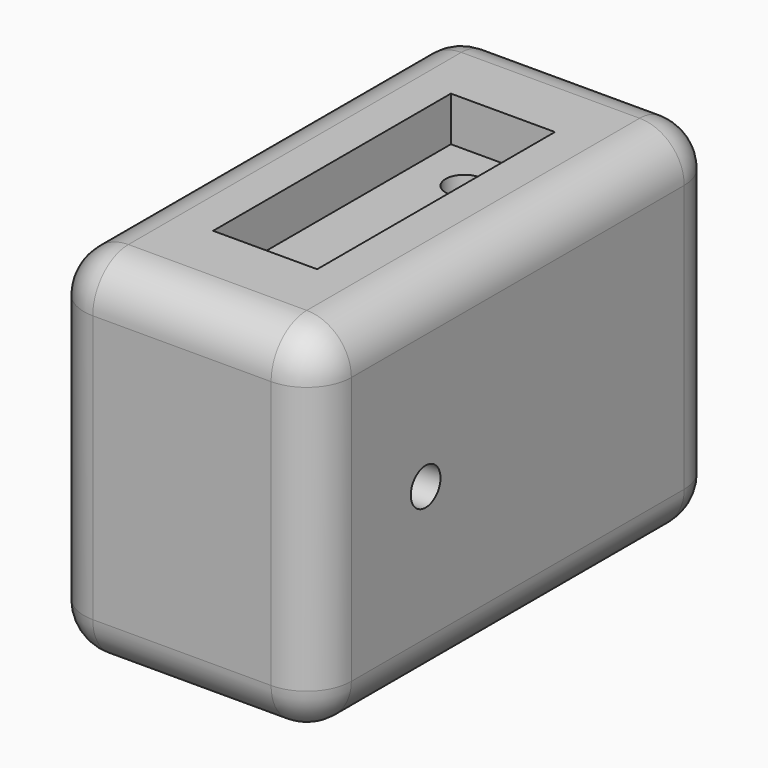
from build123d import *

# Parameters (mm, degrees)
F0_W         = 18
F0_H         = 24
F1_DEPTH     = 34
F2_W         = 25
F2_H         = 13
F2_R         = 1.25
F3_DEPTH     = 16
F4_W         = 7
F4_H         = 20
F5_DEPTH     = 3
F6_R         = 1.25
F7_DEPTH     = 4
F8_T1_DEPTH  = 28
F8_T3_DEPTH  = 18
F8_T5_DEPTH  = 12
F8_S9_W      = 3
F8_S9_H      = 3
F8_T10_DEPTH = 3
F8_S15_W     = 3
F8_S15_H     = 3
F8_T16_DEPTH = 3
F8_S21_W     = 3
F8_S21_H     = 3
F8_T22_DEPTH = 3
F8_S27_W     = 3
F8_S27_H     = 3
F8_T28_DEPTH = 3
F8_S33_W     = 3
F8_S33_H     = 3
F8_T34_DEPTH = 3
F8_S39_W     = 3
F8_S39_H     = 3
F8_T40_DEPTH = 3
F8_S45_W     = 3
F8_S45_H     = 3
F8_T46_DEPTH = 3
F8_S51_W     = 3
F8_S51_H     = 3
F8_T52_DEPTH = 3
F9_R         = 3.5
F10_DEPTH    = 19
F11_R        = 1.25
F12_DEPTH    = 18.0010001


# Not quite as in the source:
# - a fillet or chamfer that OpenCascade refuses, or shapes differently, is made with other operations: its cross-section is extruded or revolved along the edge and cut away or added


with BuildPart() as f1:
    # F0 (on Front) → F1 (new body)
    with BuildSketch(Plane.XZ):
        with Locations((-10.5989521787, -5.2339873202)):
            Rectangle(F0_W, F0_H)
    extrude(amount=F1_DEPTH)

    # F2 (on face) → F3 (cut)
    with BuildSketch(Plane(origin=(-19.5989521787, 0, 0), x_dir=(0, -1, 0), z_dir=(-1, 0, 0))):
        with Locations((17, -7.2339873202)):
            Rectangle(F2_W, F2_H)
        with Locations((2.25, -7.2339873202)):
            Circle(F2_R)
        with Locations((31.75, -7.2339873202)):
            Circle(F2_R)
    extrude(amount=-F3_DEPTH, mode=Mode.SUBTRACT)

    # F4 (on face) → F5 (cut)
    with BuildSketch(Plane.XY.offset(6.7660126798)):
        with Locations((-10.5989521787, -17)):
            Rectangle(F4_W, F4_H)
    extrude(amount=-F5_DEPTH, mode=Mode.SUBTRACT)

    # F6 (on face) → F7 (cut)
    with BuildSketch(Plane.XY.offset(3.7660126798)):
        with Locations((-10.5989521787, -10.25)):
            Circle(F6_R)
        with Locations((-10.5989521787, -23.75)):
            Circle(F6_R)
    extrude(amount=-F7_DEPTH, mode=Mode.SUBTRACT)

    # F8: fillet of radius 3 on 12 edges, made by hand

    # F8_s2 → F8_t1 (cut)
    with BuildSketch(Plane.XZ.offset(3)):
        with BuildLine():
            ThreePointArc((-19.5989521787, 3.7660126798), (-18.7202725222, 5.8873330233), (-16.5989521787, 6.7660126798))
            Line((-16.5989521787, 6.7660126798), (-19.5989521787, 6.7660126798))
            Line((-19.5989521787, 6.7660126798), (-19.5989521787, 3.7660126798))
        make_face()
        with BuildLine():
            ThreePointArc((-16.5989521787, -17.2339873202), (-18.7202725222, -16.3553076638), (-19.5989521787, -14.2339873202))
            Line((-19.5989521787, -14.2339873202), (-19.5989521787, -17.2339873202))
            Line((-19.5989521787, -17.2339873202), (-16.5989521787, -17.2339873202))
        make_face()
        with BuildLine():
            ThreePointArc((-4.5989521787, -17.2339873202), (-2.4776318351, -16.3553076638), (-1.5989521787, -14.2339873202))
            Line((-1.5989521787, -14.2339873202), (-1.5989521787, -17.2339873202))
            Line((-1.5989521787, -17.2339873202), (-4.5989521787, -17.2339873202))
        make_face()
        with BuildLine():
            ThreePointArc((-1.5989521787, 3.7660126798), (-2.4776318351, 5.8873330233), (-4.5989521787, 6.7660126798))
            Line((-4.5989521787, 6.7660126798), (-1.5989521787, 6.7660126798))
            Line((-1.5989521787, 6.7660126798), (-1.5989521787, 3.7660126798))
        make_face()
    extrude(amount=F8_T1_DEPTH, mode=Mode.SUBTRACT)

    # F8_s4 → F8_t3 (cut)
    with BuildSketch(Plane.XY.offset(-14.2339873202)):
        with BuildLine():
            ThreePointArc((-19.5989521787, -31), (-18.7202725222, -33.1213203436), (-16.5989521787, -34))
            Line((-16.5989521787, -34), (-19.5989521787, -34))
            Line((-19.5989521787, -34), (-19.5989521787, -31))
        make_face()
        with BuildLine():
            ThreePointArc((-1.5989521787, -31), (-2.4776318351, -33.1213203436), (-4.5989521787, -34))
            Line((-4.5989521787, -34), (-1.5989521787, -34))
            Line((-1.5989521787, -34), (-1.5989521787, -31))
        make_face()
        with BuildLine():
            ThreePointArc((-19.5989521787, -3), (-18.7202725222, -0.8786796564), (-16.5989521787, 0))
            Line((-16.5989521787, 0), (-19.5989521787, 0))
            Line((-19.5989521787, 0), (-19.5989521787, -3))
        make_face()
        with BuildLine():
            ThreePointArc((-1.5989521787, -3), (-2.4776318351, -0.8786796564), (-4.5989521787, 0))
            Line((-4.5989521787, 0), (-1.5989521787, 0))
            Line((-1.5989521787, 0), (-1.5989521787, -3))
        make_face()
    extrude(amount=F8_T3_DEPTH, mode=Mode.SUBTRACT)

    # F8_s6 → F8_t5 (cut)
    with BuildSketch(Plane.YZ.offset(-16.5989521787)):
        with BuildLine():
            ThreePointArc((-31, -17.2339873202), (-33.1213203436, -16.3553076638), (-34, -14.2339873202))
            Line((-34, -14.2339873202), (-34, -17.2339873202))
            Line((-34, -17.2339873202), (-31, -17.2339873202))
        make_face()
        with BuildLine():
            ThreePointArc((0, 3.7660126798), (-0.8786796564, 5.8873330233), (-3, 6.7660126798))
            Line((-3, 6.7660126798), (0, 6.7660126798))
            Line((0, 6.7660126798), (0, 3.7660126798))
        make_face()
        with BuildLine():
            ThreePointArc((-34, 3.7660126798), (-33.1213203436, 5.8873330233), (-31, 6.7660126798))
            Line((-31, 6.7660126798), (-34, 6.7660126798))
            Line((-34, 6.7660126798), (-34, 3.7660126798))
        make_face()
        with BuildLine():
            ThreePointArc((-3, -17.2339873202), (-0.8786796564, -16.3553076638), (0, -14.2339873202))
            Line((0, -14.2339873202), (0, -17.2339873202))
            Line((0, -17.2339873202), (-3, -17.2339873202))
        make_face()
    extrude(amount=F8_T5_DEPTH, mode=Mode.SUBTRACT)


with BuildPart() as f8_tool8:
    # F8_s9 → F8_t10 (new body)
    with BuildSketch(Plane.YZ.offset(-16.5989521787)):
        with Locations((-1.5, 5.2660126798)):
            Rectangle(F8_S9_W, F8_S9_H)
    extrude(amount=-F8_T10_DEPTH)

    # F8_s11 → F8_t12 (revolve, cut)
    with BuildSketch(Plane(origin=(-16.5989521787, -3, 3.7660126798), x_dir=(0, -0.7071067812, -0.7071067812), z_dir=(0, 0.7071067812, -0.7071067812))):
        with BuildLine():
            ThreePointArc((0, -3), (3, 0), (0, 3))
            Line((0, 3), (0, -3))
        make_face()
    revolve(axis=Axis((-16.5989521787, -3, 3.7660126798), (-1, 0, 0)), mode=Mode.SUBTRACT)


with BuildPart() as f1_1:
    add(f1.part)

    # F8_t7: cut F8_tool8
    add(f8_tool8.part, mode=Mode.SUBTRACT)


with BuildPart() as f8_tool14:
    # F8_s15 → F8_t16 (new body)
    with BuildSketch(Plane.YZ.offset(-16.5989521787)):
        with Locations((-32.5, 5.2660126798)):
            Rectangle(F8_S15_W, F8_S15_H)
    extrude(amount=-F8_T16_DEPTH)

    # F8_s17 → F8_t18 (revolve, cut)
    with BuildSketch(Plane(origin=(-16.5989521787, -31, 3.7660126798), x_dir=(0, 0.7071067812, -0.7071067812), z_dir=(0, 0.7071067812, 0.7071067812))):
        with BuildLine():
            ThreePointArc((0, -3), (3, 0), (0, 3))
            Line((0, 3), (0, -3))
        make_face()
    revolve(axis=Axis((-16.5989521787, -31, 3.7660126798), (-1, 0, 0)), mode=Mode.SUBTRACT)


with BuildPart() as f1_2:
    add(f1_1.part)

    # F8_t13: cut F8_tool14
    add(f8_tool14.part, mode=Mode.SUBTRACT)


with BuildPart() as f8_tool20:
    # F8_s21 → F8_t22 (new body)
    with BuildSketch(Plane.XY.offset(-14.2339873202)):
        with Locations((-18.0989521787, -32.5)):
            Rectangle(F8_S21_W, F8_S21_H)
    extrude(amount=-F8_T22_DEPTH)

    # F8_s23 → F8_t24 (revolve, cut)
    with BuildSketch(Plane(origin=(-16.5989521787, -31, -14.2339873202), x_dir=(0.7071067812, 0.7071067812, 0), z_dir=(-0.7071067812, 0.7071067812, 0))):
        with BuildLine():
            ThreePointArc((0, -3), (3, 0), (0, 3))
            Line((0, 3), (0, -3))
        make_face()
    revolve(axis=Axis((-16.5989521787, -31, -14.2339873202), (0, 0, -1)), mode=Mode.SUBTRACT)


with BuildPart() as f1_3:
    add(f1_2.part)

    # F8_t19: cut F8_tool20
    add(f8_tool20.part, mode=Mode.SUBTRACT)


with BuildPart() as f8_tool26:
    # F8_s27 → F8_t28 (new body)
    with BuildSketch(Plane.XY.offset(-14.2339873202)):
        with Locations((-3.0989521787, -32.5)):
            Rectangle(F8_S27_W, F8_S27_H)
    extrude(amount=-F8_T28_DEPTH)

    # F8_s29 → F8_t30 (revolve, cut)
    with BuildSketch(Plane(origin=(-4.5989521787, -31, -14.2339873202), x_dir=(-0.7071067812, 0.7071067812, 0), z_dir=(-0.7071067812, -0.7071067812, 0))):
        with BuildLine():
            ThreePointArc((0, -3), (3, 0), (0, 3))
            Line((0, 3), (0, -3))
        make_face()
    revolve(axis=Axis((-4.5989521787, -31, -14.2339873202), (0, 0, -1)), mode=Mode.SUBTRACT)


with BuildPart() as f1_4:
    add(f1_3.part)

    # F8_t25: cut F8_tool26
    add(f8_tool26.part, mode=Mode.SUBTRACT)


with BuildPart() as f8_tool32:
    # F8_s33 → F8_t34 (new body)
    with BuildSketch(Plane.YZ.offset(-4.5989521787)):
        with Locations((-32.5, 5.2660126798)):
            Rectangle(F8_S33_W, F8_S33_H)
    extrude(amount=F8_T34_DEPTH)

    # F8_s35 → F8_t36 (revolve, cut)
    with BuildSketch(Plane(origin=(-4.5989521787, -31, 3.7660126798), x_dir=(0, 0.7071067812, -0.7071067812), z_dir=(0, -0.7071067812, -0.7071067812))):
        with BuildLine():
            ThreePointArc((0, -3), (3, 0), (0, 3))
            Line((0, 3), (0, -3))
        make_face()
    revolve(axis=Axis((-4.5989521787, -31, 3.7660126798), (1, 0, 0)), mode=Mode.SUBTRACT)


with BuildPart() as f1_5:
    add(f1_4.part)

    # F8_t31: cut F8_tool32
    add(f8_tool32.part, mode=Mode.SUBTRACT)


with BuildPart() as f8_tool38:
    # F8_s39 → F8_t40 (new body)
    with BuildSketch(Plane.XY.offset(-14.2339873202)):
        with Locations((-18.0989521787, -1.5)):
            Rectangle(F8_S39_W, F8_S39_H)
    extrude(amount=-F8_T40_DEPTH)

    # F8_s41 → F8_t42 (revolve, cut)
    with BuildSketch(Plane(origin=(-16.5989521787, -3, -14.2339873202), x_dir=(0.7071067812, -0.7071067812, 0), z_dir=(0.7071067812, 0.7071067812, 0))):
        with BuildLine():
            ThreePointArc((0, -3), (3, 0), (0, 3))
            Line((0, 3), (0, -3))
        make_face()
    revolve(axis=Axis((-16.5989521787, -3, -14.2339873202), (0, 0, -1)), mode=Mode.SUBTRACT)


with BuildPart() as f1_6:
    add(f1_5.part)

    # F8_t37: cut F8_tool38
    add(f8_tool38.part, mode=Mode.SUBTRACT)


with BuildPart() as f8_tool44:
    # F8_s45 → F8_t46 (new body)
    with BuildSketch(Plane.XY.offset(-14.2339873202)):
        with Locations((-3.0989521787, -1.5)):
            Rectangle(F8_S45_W, F8_S45_H)
    extrude(amount=-F8_T46_DEPTH)

    # F8_s47 → F8_t48 (revolve, cut)
    with BuildSketch(Plane(origin=(-4.5989521787, -3, -14.2339873202), x_dir=(-0.7071067812, -0.7071067812, 0), z_dir=(0.7071067812, -0.7071067812, 0))):
        with BuildLine():
            ThreePointArc((0, -3), (3, 0), (0, 3))
            Line((0, 3), (0, -3))
        make_face()
    revolve(axis=Axis((-4.5989521787, -3, -14.2339873202), (0, 0, -1)), mode=Mode.SUBTRACT)


with BuildPart() as f1_7:
    add(f1_6.part)

    # F8_t43: cut F8_tool44
    add(f8_tool44.part, mode=Mode.SUBTRACT)


with BuildPart() as f8_tool50:
    # F8_s51 → F8_t52 (new body)
    with BuildSketch(Plane.YZ.offset(-4.5989521787)):
        with Locations((-1.5, 5.2660126798)):
            Rectangle(F8_S51_W, F8_S51_H)
    extrude(amount=F8_T52_DEPTH)

    # F8_s53 → F8_t54 (revolve, cut)
    with BuildSketch(Plane(origin=(-4.5989521787, -3, 3.7660126798), x_dir=(0, -0.7071067812, -0.7071067812), z_dir=(0, -0.7071067812, 0.7071067812))):
        with BuildLine():
            ThreePointArc((0, -3), (3, 0), (0, 3))
            Line((0, 3), (0, -3))
        make_face()
    revolve(axis=Axis((-4.5989521787, -3, 3.7660126798), (1, 0, 0)), mode=Mode.SUBTRACT)


with BuildPart() as f1_8:
    add(f1_7.part)

    # F8_t49: cut F8_tool50
    add(f8_tool50.part, mode=Mode.SUBTRACT)

    # F9 (on face) → F10 (cut)
    with BuildSketch(Plane(origin=(0, 0, -17.2339873202), x_dir=(1, 0, 0), z_dir=(0, 0, -1))):
        with Locations((-10.5989521787, 10.5)):
            Circle(F9_R)
        with Locations((-10.5989521787, 23.5)):
            Circle(F9_R)
    extrude(amount=-F10_DEPTH, mode=Mode.SUBTRACT)

    # F11 (on face) → F12 (cut, through all)
    with BuildSketch(Plane.YZ.offset(-1.5989521787)):
        with Locations((-24.75, -5.2339873202)):
            Circle(F11_R)
    extrude(amount=-F12_DEPTH, mode=Mode.SUBTRACT)


solid = f1_8.part
